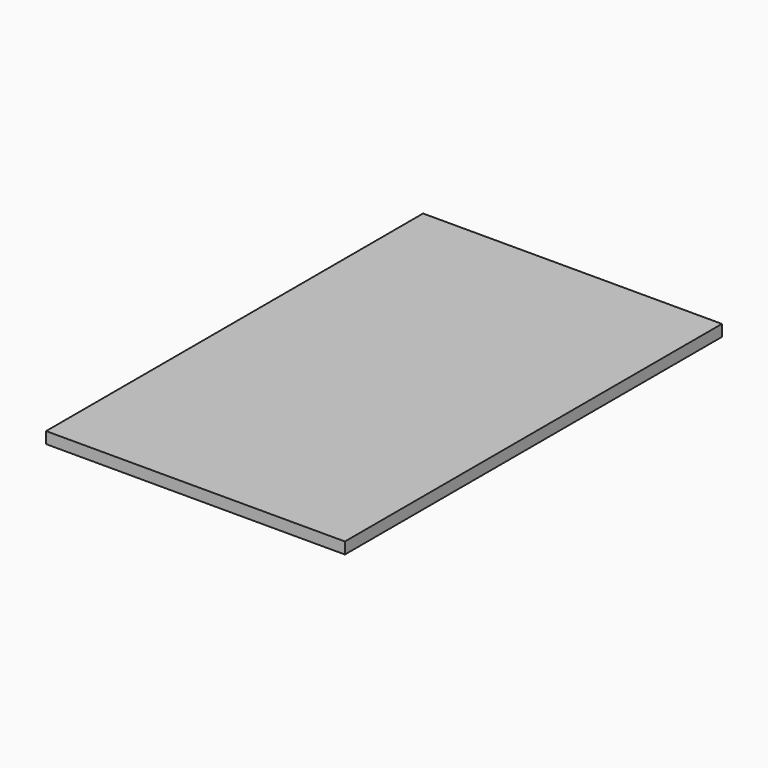
from build123d import *

# Parameters (mm, degrees)
F0_W     = 660.4
F0_H     = 1041.4
F1_DEPTH = 25.4


# Not quite as in the source:
# - a feature names something its author has since deleted; it is built from what else it names


with BuildPart() as f1:
    # F0 (on Top) → F1 (new body)
    with BuildSketch(Plane.XY):
        Rectangle(F0_W, F0_H)
    extrude(amount=F1_DEPTH)


solid = f1.part
